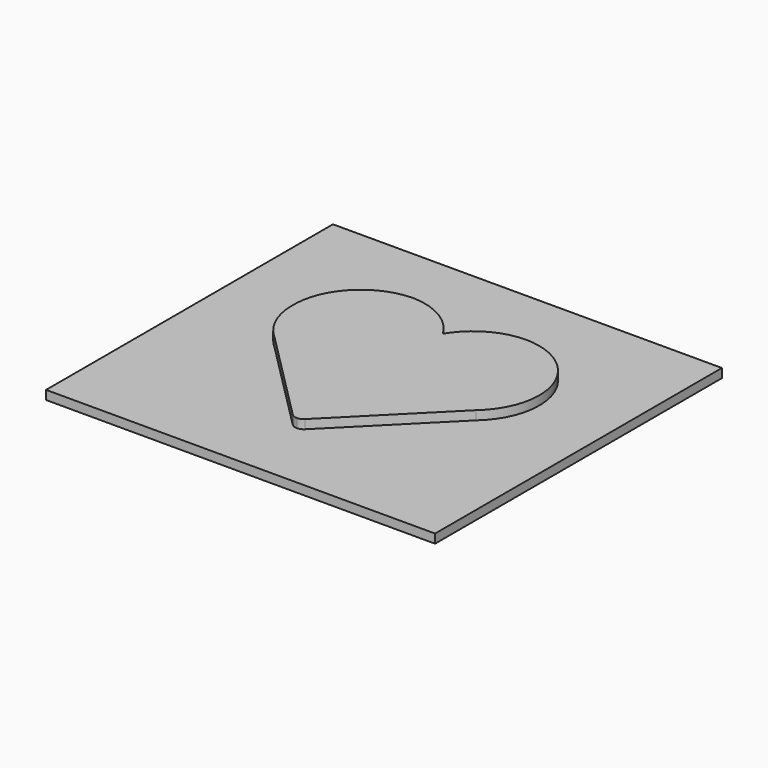
from build123d import *

# Parameters (mm, degrees)
F0_W      = 137.7741502185
F0_H      = 127
F1_DEPTH  = 6.35
F1_FACE_W = 137.7741502185
F1_FACE_H = 127
F2_DEPTH  = 3.175


# Not quite as in the source:
# - a length typed as a fraction of an inch, garbled in the dataset ("3 / 203.2 mm" for 3/8 in), is restored


with BuildPart() as f1:
    # F0 (on Top) → F1 (new body)
    with BuildSketch(Plane.XY):
        Rectangle(F0_W, F0_H)
        with BuildLine():
            add(Edge.make_bspline(
                [(43.4870751092, 14.3433300558), (43.4870751092, 27.462876741), (32.8514196183, 38.0979859262), (19.7318729331, 38.0979859262)],
                knots=[0, 0, 0, 0, 1, 1, 1, 1], degree=3))
            add(Edge.make_bspline(
                [(35.3328363694, -3.5415767003), (40.3215229837, 0.8101175052), (43.4870751092, 7.2004637855), (43.4870751092, 14.3433300558)],
                knots=[0, 0, 0, 0, 1, 1, 1, 1], degree=3))
            Line((35.3328363694, -3.5415767003), (1.7854201908, -37.2041767762))
            add(Edge.make_bspline(
                [(-0.3831377338, -38.1), (0.4300700378, -38.1007554216), (1.2100121742, -37.7785167454), (1.7854201908, -37.2041767762)],
                knots=[0, 0, 0, 0, 1, 1, 1, 1], degree=3))
            add(Edge.make_bspline(
                [(-2.5508625567, -37.2021627024), (-1.9759883158, -37.7770369433), (-1.1963458563, -38.1), (-0.3831377338, -38.1)],
                knots=[0, 0, 0, 0, 1, 1, 1, 1], degree=3))
            Line((-2.5508625567, -37.2021627024), (-35.3333666072, -4.280217526))
            add(Edge.make_bspline(
                [(-43.4870751092, 13.6046892301), (-43.4870751092, 6.4618229599), (-40.3218925434, 0.0714766795), (-35.3333666072, -4.280217526)],
                knots=[0, 0, 0, 0, 1, 1, 1, 1], degree=3))
            add(Edge.make_bspline(
                [(-20.4995127814, 38.1), (-33.6124722867, 37.6843099249), (-43.9027651844, 26.7176487354), (-43.4870751092, 13.6046892301)],
                knots=[0, 0, 0, 0, 1, 1, 1, 1], degree=3))
            add(Edge.make_bspline(
                [(-0.3831377338, 26.5499493108), (-4.4942474015, 33.3906018689), (-11.9332866772, 38.0146472183), (-20.4995127814, 38.1)],
                knots=[0, 0, 0, 0, 1, 1, 1, 1], degree=3))
            add(Edge.make_bspline(
                [(19.7318729331, 38.0979859262), (11.16547776, 38.0134786667), (3.7291785921, 33.3902005219), (-0.3831377338, 26.5499493108)],
                knots=[0, 0, 0, 0, 1, 1, 1, 1], degree=3))
        make_face(mode=Mode.SUBTRACT)
        with BuildLine():
            add(Edge.make_bspline(
                [(35.3328363694, -3.5415767003), (40.3215229837, 0.8101175052), (43.4870751092, 7.2004637855), (43.4870751092, 14.3433300558)],
                knots=[0, 0, 0, 0, 1, 1, 1, 1], degree=3))
            add(Edge.make_bspline(
                [(43.4870751092, 14.3433300558), (43.4870751092, 27.462876741), (32.8514196183, 38.0979859262), (19.7318729331, 38.0979859262)],
                knots=[0, 0, 0, 0, 1, 1, 1, 1], degree=3))
            add(Edge.make_bspline(
                [(19.7318729331, 38.0979859262), (11.16547776, 38.0134786667), (3.7291785921, 33.3902005219), (-0.3831377338, 26.5499493108)],
                knots=[0, 0, 0, 0, 1, 1, 1, 1], degree=3))
            add(Edge.make_bspline(
                [(-0.3831377338, 26.5499493108), (-4.4942474015, 33.3906018689), (-11.9332866772, 38.0146472183), (-20.4995127814, 38.1)],
                knots=[0, 0, 0, 0, 1, 1, 1, 1], degree=3))
            add(Edge.make_bspline(
                [(-20.4995127814, 38.1), (-33.6124722867, 37.6843099249), (-43.9027651844, 26.7176487354), (-43.4870751092, 13.6046892301)],
                knots=[0, 0, 0, 0, 1, 1, 1, 1], degree=3))
            add(Edge.make_bspline(
                [(-43.4870751092, 13.6046892301), (-43.4870751092, 6.4618229599), (-40.3218925434, 0.0714766795), (-35.3333666072, -4.280217526)],
                knots=[0, 0, 0, 0, 1, 1, 1, 1], degree=3))
            Line((-35.3333666072, -4.280217526), (-2.5508625567, -37.2021627024))
            add(Edge.make_bspline(
                [(-2.5508625567, -37.2021627024), (-1.9759883158, -37.7770369433), (-1.1963458563, -38.1), (-0.3831377338, -38.1)],
                knots=[0, 0, 0, 0, 1, 1, 1, 1], degree=3))
            add(Edge.make_bspline(
                [(-0.3831377338, -38.1), (0.4300700378, -38.1007554216), (1.2100121742, -37.7785167454), (1.7854201908, -37.2041767762)],
                knots=[0, 0, 0, 0, 1, 1, 1, 1], degree=3))
            Line((1.7854201908, -37.2041767762), (35.3328363694, -3.5415767003))
        make_face()
    extrude(amount=-F1_DEPTH)

    # F0 (on Top) + F1_face (on face) → F2 (cut)
    with BuildSketch(Plane.XY):
        Rectangle(F0_W, F0_H)
        with BuildLine():
            add(Edge.make_bspline(
                [(43.4870751092, 14.3433300558), (43.4870751092, 27.462876741), (32.8514196183, 38.0979859262), (19.7318729331, 38.0979859262)],
                knots=[0, 0, 0, 0, 1, 1, 1, 1], degree=3))
            add(Edge.make_bspline(
                [(35.3328363694, -3.5415767003), (40.3215229837, 0.8101175052), (43.4870751092, 7.2004637855), (43.4870751092, 14.3433300558)],
                knots=[0, 0, 0, 0, 1, 1, 1, 1], degree=3))
            Line((35.3328363694, -3.5415767003), (1.7854201908, -37.2041767762))
            add(Edge.make_bspline(
                [(-0.3831377338, -38.1), (0.4300700378, -38.1007554216), (1.2100121742, -37.7785167454), (1.7854201908, -37.2041767762)],
                knots=[0, 0, 0, 0, 1, 1, 1, 1], degree=3))
            add(Edge.make_bspline(
                [(-2.5508625567, -37.2021627024), (-1.9759883158, -37.7770369433), (-1.1963458563, -38.1), (-0.3831377338, -38.1)],
                knots=[0, 0, 0, 0, 1, 1, 1, 1], degree=3))
            Line((-2.5508625567, -37.2021627024), (-35.3333666072, -4.280217526))
            add(Edge.make_bspline(
                [(-43.4870751092, 13.6046892301), (-43.4870751092, 6.4618229599), (-40.3218925434, 0.0714766795), (-35.3333666072, -4.280217526)],
                knots=[0, 0, 0, 0, 1, 1, 1, 1], degree=3))
            add(Edge.make_bspline(
                [(-20.4995127814, 38.1), (-33.6124722867, 37.6843099249), (-43.9027651844, 26.7176487354), (-43.4870751092, 13.6046892301)],
                knots=[0, 0, 0, 0, 1, 1, 1, 1], degree=3))
            add(Edge.make_bspline(
                [(-0.3831377338, 26.5499493108), (-4.4942474015, 33.3906018689), (-11.9332866772, 38.0146472183), (-20.4995127814, 38.1)],
                knots=[0, 0, 0, 0, 1, 1, 1, 1], degree=3))
            add(Edge.make_bspline(
                [(19.7318729331, 38.0979859262), (11.16547776, 38.0134786667), (3.7291785921, 33.3902005219), (-0.3831377338, 26.5499493108)],
                knots=[0, 0, 0, 0, 1, 1, 1, 1], degree=3))
        make_face(mode=Mode.SUBTRACT)
    with BuildSketch(Plane(origin=(0, 0, -6.35), x_dir=(1, 0, 0), z_dir=(0, 0, -1))):
        Rectangle(F1_FACE_W, F1_FACE_H)
    extrude(amount=-F2_DEPTH, dir=(0, 0, 1), mode=Mode.SUBTRACT)


solid = f1.part
